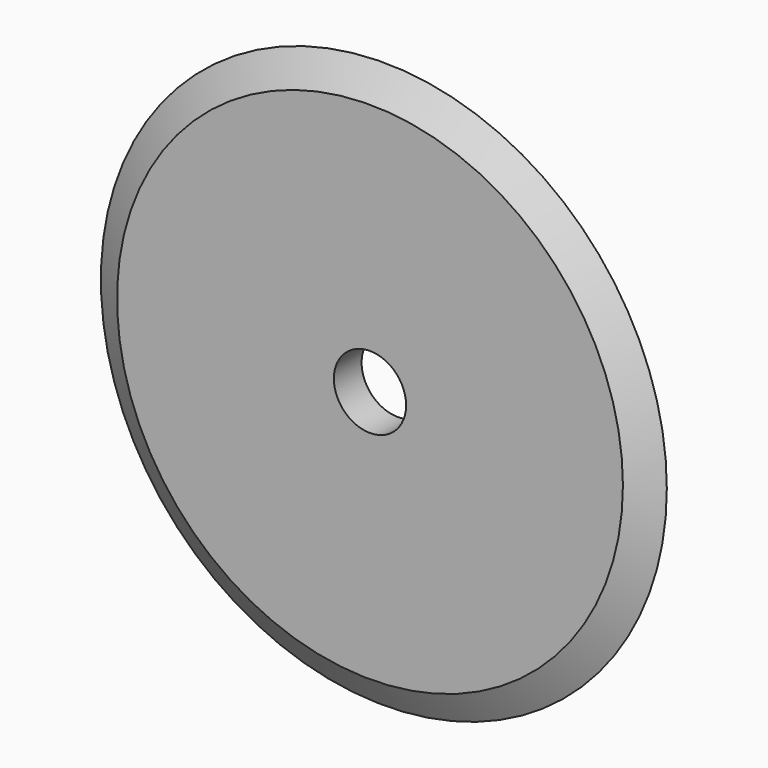
from build123d import *

# Parameters (mm, degrees)
F0_R     = 25.4
F0_R_2   = 3.175
F1_DEPTH = 3.048
F2_SIZE2 = 1.8330871047
F2_SIZE  = 3.175


# Not quite as in the source:
# - a fillet or chamfer that OpenCascade refuses, or shapes differently, is made with other operations: its cross-section is extruded or revolved along the edge and cut away or added


with BuildPart() as f1:
    # F0 (on Front) → F1 (new body)
    with BuildSketch(Plane.XZ):
        Circle(F0_R)
        Circle(F0_R_2, mode=Mode.SUBTRACT)
    extrude(amount=F1_DEPTH)

    # F2
    f2_edges = [f1.edges().sort_by_distance(p)[0] for p in [
        (-25.4, -3.048, 0),
    ]]
    f2_side = f1.faces().sort_by_distance((-24.68158, -3.048, 0))[0]
    chamfer(f2_edges, length=F2_SIZE, length2=F2_SIZE2, reference=f2_side)

    # F3: chamfer of 3.175 x 1.8330871047 on 1 edges, made by hand

    # F3_s1 → F3_t2 (revolve, cut)
    with BuildSketch(Plane.XY):
        Polygon((25.4, -1.8330871047), (22.225, 0), (25.4, 0), align=None)
    revolve(axis=Axis((0, 0, 0), (0, -1, 0)), mode=Mode.SUBTRACT)


solid = f1.part
